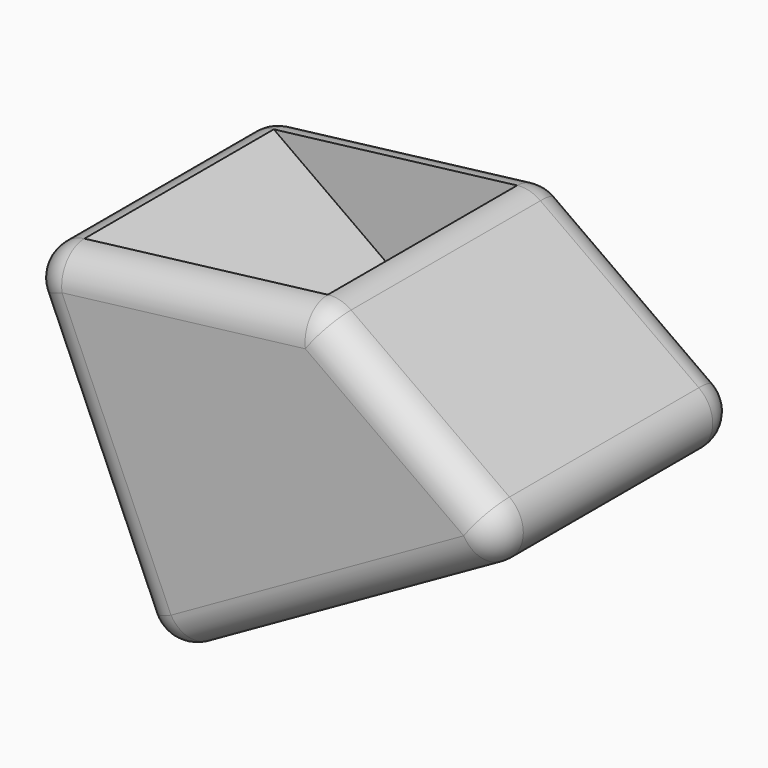
from build123d import *

# Parameters (mm, degrees)
F1_DEPTH   = 46.482
F3_R       = 5.08
F1_FACE1_W = 37.6294337092
F1_FACE1_H = 36.322


# Not quite as in the source:
# - a feature of the source that left no trace in its solid (it failed there, or was rolled back) is left out


with BuildPart() as f1:
    # F0 (on Front) → F1 (new body)
    with BuildSketch(Plane.XZ):
        Polygon((-2.8179630172, 51.4278113842), (-48.9117763937, 45.7918867469), (-27.1732080728, -3.7237356883), (29.5886062086, 28.2802637666), align=None)
    extrude(amount=F1_DEPTH)

    # F3
    f3_edges = [f1.edges().sort_by_distance(p)[0] for p in [
        (-2.817963, -23.241, 51.427811),
        (-48.911776, -23.241, 45.791887),
        (-25.86487, 0, 48.609849),
        (-25.86487, -46.482, 48.609849),
        (-38.042492, 0, 21.034076),
        (1.207699, 0, 12.278264),
        (13.385322, 0, 39.854038),
        (-27.173208, -23.241, -3.723736),
        (29.588606, -23.241, 28.280264),
        (1.207699, -46.482, 12.278264),
        (-38.042492, -46.482, 21.034076),
        (13.385322, -46.482, 39.854038),
    ]]
    fillet(f3_edges, radius=F3_R)

    # F4: sweep along a path in F4_path
    with BuildLine(Plane(origin=(23.0940504855, -41.402, 32.9192317736), x_dir=(0.8137334929, 0, -0.5812381633), z_dir=(-0.5812381633, 0, -0.8137334929))) as f4_path:
        Line((0, 0), (-29.867419561, 0))
    # F1_face1 (on face) → F4 (sweep, cut)
    with BuildSketch(Plane(origin=(-25.8648697054, -23.241, 48.6098490655), x_dir=(1, 0, 0), z_dir=(-0.1213668794, 0, 0.9926077174))):
        with Locations((2.4278813649, 0)):
            Rectangle(F1_FACE1_W, F1_FACE1_H)
    sweep(path=f4_path.line, mode=Mode.SUBTRACT)


solid = f1.part
